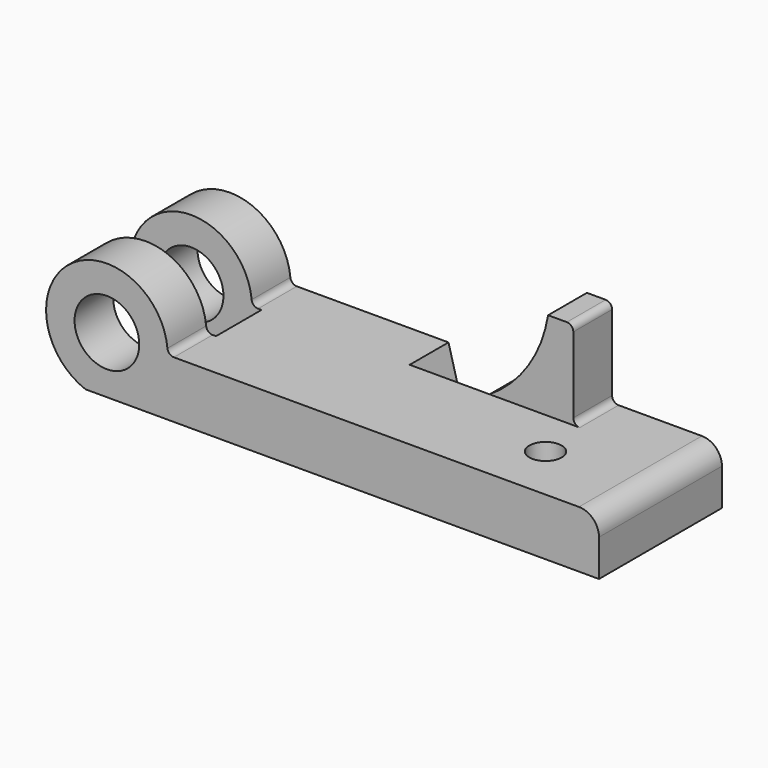
from build123d import *
from build123d import SkipClean  # not in build123d's __all__

# Parameters (mm, degrees)
F0_W          = 216.5604
F0_H          = 60.325
F1_DEPTH      = 11.176
F2_R          = 23.876
F2_R_2        = 12.7
F3_DEPTH      = 60.325
F5_DEPTH      = 60.326
F6_W          = 1.016
F6_H          = 60.325
F6_W_2        = 60.7332959771
F6_H_2        = 22.3266
F6_R          = 6.35
F7_DEPTH      = 22.353
F7_DEPTH_BACK = 23.877
F10_DEPTH     = 19.05
F11_DEPTH     = 19.05
F12_R         = 2.54
F13_R         = 7.874


# Not quite as in the source:
# - after a boolean that leaves OpenCascade's solid faulty, fix() repairs it


with BuildPart() as f1:
    # F0 (on Top) → F1 (new body, symmetric)
    with BuildSketch(Plane.XY):
        Rectangle(F0_W, F0_H)
    extrude(amount=F1_DEPTH, both=True)

    # F2 (on face) → F3 (join, through all)
    with BuildSketch(Plane.XZ.offset(30.1625)):
        with Locations((-85.9282, 11.176)):
            Circle(F2_R)
        with Locations((-85.9282, 11.176)):
            Circle(F2_R_2, mode=Mode.SUBTRACT)
    extrude(amount=-F3_DEPTH)

    # F4 (on face) → F5 (cut, through all)
    with BuildSketch(Plane.XZ.offset(30.1625)):
        with BuildLine():
            Line((-108.2802, -11.176), (-94.3217375141, -11.176))
            ThreePointArc((-94.3217375141, -11.176), (-102.8110815076, -5.7068815076), (-108.2802, 2.7824624859))
            Line((-108.2802, 2.7824624859), (-108.2802, -11.176))
        make_face()
        with BuildLine():
            Line((-77.5346624859, -11.176), (-94.3217375141, -11.176))
            ThreePointArc((-94.3217375141, -11.176), (-85.9282, -12.7), (-77.5346624859, -11.176))
        make_face()
        with BuildLine():
            ThreePointArc((-98.6282, 11.176), (-85.9282, -1.524), (-73.2282, 11.176))
            Line((-73.2282, 11.176), (-98.6282, 11.176))
        make_face()
    with SkipClean():  # cleaning this boolean's faces spoils the solid; the shape is the same uncleaned
        extrude(amount=-F5_DEPTH, mode=Mode.SUBTRACT)

    # F6 (on face) → F7 (cut, two sides)
    with BuildSketch(Plane.XY.offset(11.176)) as f7_sk:
        with Locations((107.7722, 0)):
            Rectangle(F6_W, F6_H)
        with Locations((-88.6705182493, 0)):
            Rectangle(F6_W_2, F6_H_2)
        with Locations((68.4022, -7.8105)):
            Circle(F6_R)
    with SkipClean():  # cleaning this boolean's faces spoils the solid; the shape is the same uncleaned
        extrude(amount=-F7_DEPTH, mode=Mode.SUBTRACT)
        extrude(f7_sk.sketch, amount=F7_DEPTH_BACK, mode=Mode.SUBTRACT)

    # F8 (on face) → F10 (cut)
    with BuildSketch(Plane(origin=(0, 30.1625, 0), x_dir=(-1, 0, 0), z_dir=(0, 1, 0))):
        Polygon((0.0762, 11.176), (-31.3182, 11.176), (-31.3182, -11.176), (-5.9182, -11.176), align=None)
    extrude(amount=-F10_DEPTH, mode=Mode.SUBTRACT)

    add(f1.part.fix(), mode=Mode.REPLACE)

    # F9 (on face) → F11 (join)
    with BuildSketch(Plane(origin=(0, 30.1625, 0), x_dir=(-1, 0, 0), z_dir=(0, 1, 0))):
        Polygon((-64.1604, 45.974), (-64.1604, -11.176), (-54.2544, -11.176), (-54.2544, 11.176), (-54.2544, 45.974), align=None)
        with BuildLine():
            Line((-54.2544, 45.974), (-54.2544, 11.176))
            Line((-54.2544, 11.176), (-31.3182, 11.176))
            ThreePointArc((-31.3182, 11.176), (-46.5191498234, 26.114588766), (-54.2544, 45.974))
        make_face()
    extrude(amount=-F11_DEPTH)

    add(f1.part.fix(), mode=Mode.REPLACE)

    # F12
    f12_edges = [f1.edges().sort_by_distance(p)[0] for p in [
        (-62.0522, 20.6629, 11.176),
        (-62.0522, -20.6629, 11.176),
        (64.1604, 20.6375, 45.974),
        (64.1604, 20.6375, 11.176),
    ]]
    fillet(f12_edges, radius=F12_R)

    # F13
    f13_edges = [f1.edges().sort_by_distance(p)[0] for p in [
        (107.2642, 0, 11.176),
    ]]
    fillet(f13_edges, radius=F13_R)


solid = f1.part
